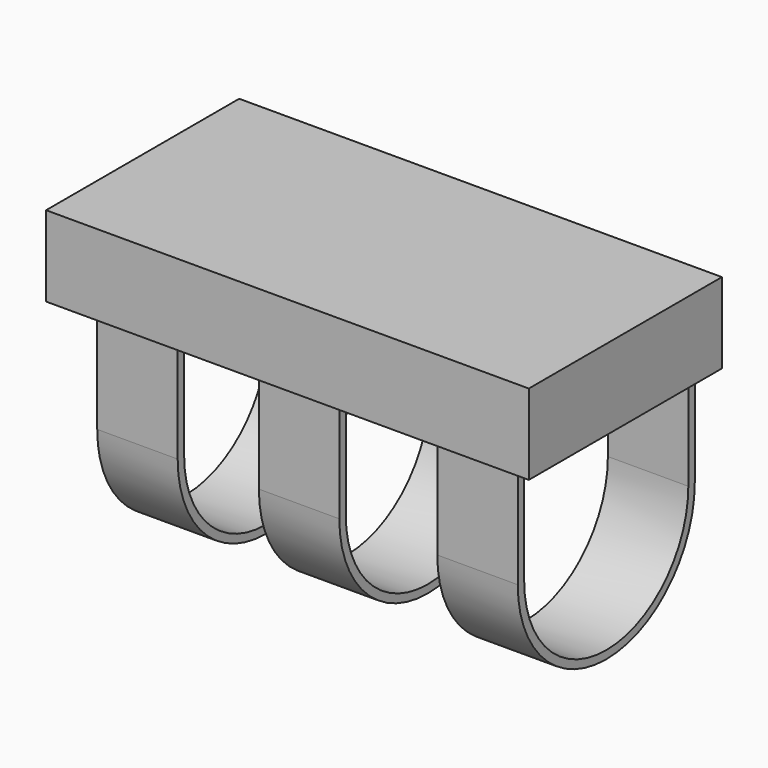
from build123d import *

# Parameters (mm, degrees)
F0_W      = 120
F0_H      = 60
F1_DEPTH  = 20
F2_W      = 20
F2_H      = 2
F3_DEPTH  = 25.5
F4_W      = 20
F4_H      = 2
F3_FACE_W = 20
F3_FACE_H = 2
F5_ANGLE  = 180


# Not quite as in the source:
# - a feature names something its author has since deleted; it is built from what else it names


with BuildPart() as f1:
    # F0 (on Top) → F1 (new body)
    with BuildSketch(Plane.XY):
        Rectangle(F0_W, F0_H)
    extrude(amount=F1_DEPTH)

    # F2 (on face) → F3 (join)
    with BuildSketch(Plane(origin=(0, 0, 0), x_dir=(1, 0, 0), z_dir=(0, 0, -1))):
        with Locations((-39.2824916542, 26.5)):
            Rectangle(F2_W, F2_H)
        with Locations((-39.2824916542, -26.5)):
            Rectangle(F2_W, F2_H)
        with Locations((0.8980135992, 26.5)):
            Rectangle(F2_W, F2_H)
        with Locations((0.8980135992, -26.5)):
            Rectangle(F2_W, F2_H)
        with Locations((45.2481971681, 26.5)):
            Rectangle(F2_W, F2_H)
        with Locations((45.2481971681, -26.5)):
            Rectangle(F2_W, F2_H)
    extrude(amount=F3_DEPTH)

    # F4 (on face) + F3_face (on face) → F5 (revolve)
    with BuildSketch(Plane(origin=(0, 0, -25.5), x_dir=(1, 0, 0), z_dir=(0, 0, -1))):
        with Locations((-39.2824916542, 26.5)):
            Rectangle(F4_W, F4_H)
    with BuildSketch(Plane(origin=(-39.2824916542, -26.5, -25.5), x_dir=(1, 0, 0), z_dir=(0, 0, -1))):
        with Locations((40.1805052534, 0)):
            Rectangle(F3_FACE_W, F3_FACE_H)
        with Locations((84.5306888223, 0)):
            Rectangle(F3_FACE_W, F3_FACE_H)
    revolve(axis=Axis((1.9900724292, 0, -25.5), (1, 0, 0)), revolution_arc=F5_ANGLE)


solid = f1.part
